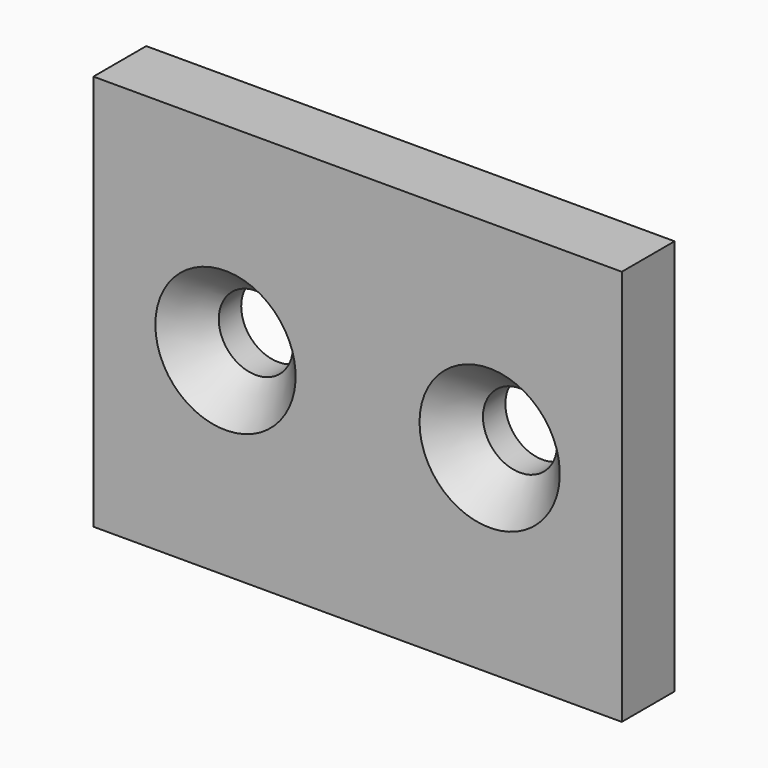
from build123d import *

# Parameters (mm, degrees)
F0_W           = 50.8
F0_H           = 38.1
F1_DEPTH       = 6.35
F3_D           = 7.1374
F3_CSINK_D     = 13.4874
F3_CSINK_ANGLE = 82


with BuildPart() as f1:
    # F0 (on Front) → F1 (new body)
    with BuildSketch(Plane.XZ):
        with Locations((25.4, 19.05)):
            Rectangle(F0_W, F0_H)
    extrude(amount=F1_DEPTH)

    # F3 (through all)
    with Locations(Plane.XZ.offset(6.35)):
        with Locations((12.7, 19.05), (38.1, 19.05)):
            CounterSinkHole(F3_D / 2, F3_CSINK_D / 2, counter_sink_angle=F3_CSINK_ANGLE)


solid = f1.part
